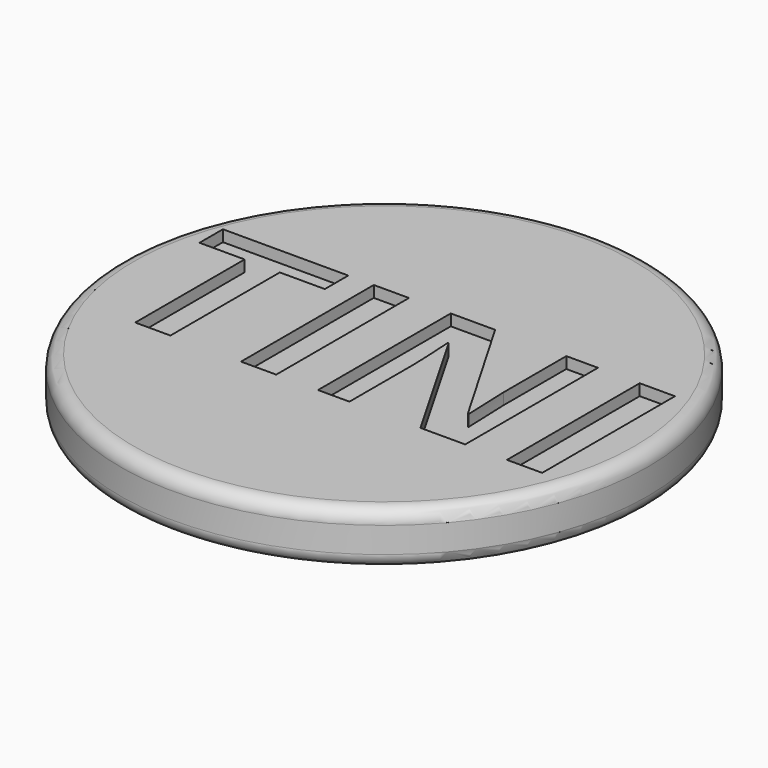
from build123d import *

# Parameters (mm, degrees)
F0_R         = 11.605
F1_DEPTH     = 1.165
F2_R         = 0.6
F3_TEXT_SIZE = 10.2209082728
F4_DEPTH     = 0.5
F5_TEXT_SIZE = 10.5460634462
F6_DEPTH     = 0.5


# Not quite as in the source:
# - Text() gives the source's letters only with a copy of the font that has no kerning and outlines rounded to 1/6400 em; it was checked with that copy


with BuildPart() as f1:
    # F0 (on Top) → F1 (new body, symmetric)
    with BuildSketch(Plane.XY):
        Circle(F0_R)
    extrude(amount=F1_DEPTH, both=True)

    # F2
    f2_edges = [f1.edges().sort_by_distance(p)[0] for p in [
        (-11.605, 0, -1.165),
        (11.605, 0, 0),
        (-11.605, 0, 1.165),
    ]]
    fillet(f2_edges, radius=F2_R)

    # F3 (on face) → F4 (cut)
    with BuildSketch(Plane.XY.offset(1.165)):
        with Locations((-10.3128451183, -3.5177975779)):
            Text('TINI', F3_TEXT_SIZE, font='Open Sans', font_style=FontStyle.BOLD, text_align=(TextAlign.LEFT, TextAlign.BOTTOM))
    extrude(amount=-F4_DEPTH, mode=Mode.SUBTRACT)

    # F5 (on face) → F6 (cut)
    with BuildSketch(Plane(origin=(0, 0, -1.165), x_dir=(1, 0, 0), z_dir=(0, 0, -1))):
        with Locations((-10.3293747988, -3.7965828406)):
            Text('TUT', F5_TEXT_SIZE, font='Open Sans', font_style=FontStyle.BOLD, text_align=(TextAlign.LEFT, TextAlign.BOTTOM))
    extrude(amount=-F6_DEPTH, mode=Mode.SUBTRACT)


solid = f1.part
